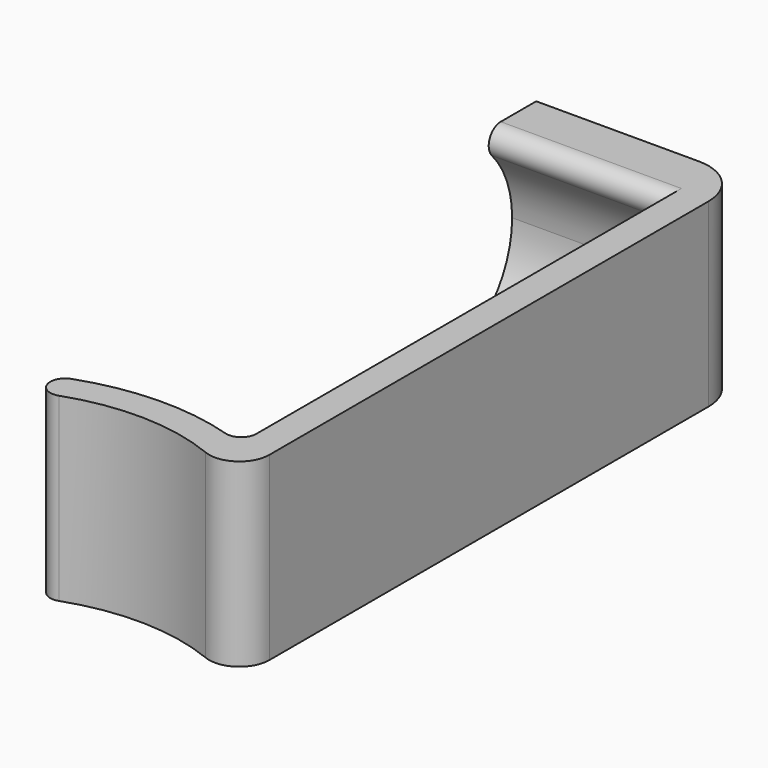
from build123d import *

# Parameters (mm, degrees)
F2_DEPTH    = 9.525
F3_DEPTH    = 19.05
F4_T1_DEPTH = 31.861787518
F5_R        = 5.08


# Not quite as in the source:
# - a fillet or chamfer that OpenCascade refuses, or shapes differently, is made with other operations: its cross-section is extruded or revolved along the edge and cut away or added


with BuildPart() as f2:
    # F0 (on Top) → F2 (new body, symmetric)
    with BuildSketch(Plane.XY):
        with BuildLine():
            Line((0, 3.175), (0, 0))
            Line((0, 0), (19.05, 0))
            Line((19.05, 0), (19.05, -57.5181780653))
            ThreePointArc((19.05, -57.5181780653), (18.4056155347, -58.7951625359), (16.9955882353, -59.0354617085))
            ThreePointArc((16.9955882353, -59.0354617085), (9.0004674941, -57.9174166081), (1.0583333333, -59.3646503438))
            ThreePointArc((1.0583333333, -59.3646503438), (0.2913116778, -59.944816145), (0, -60.8613596973))
            ThreePointArc((0, -60.8613596973), (0.6709564477, -62.1575480195), (2.1166666667, -62.3580690508))
            ThreePointArc((2.1166666667, -62.3580690508), (10.0201305345, -61.0925159656), (17.859375, -62.708873578))
            ThreePointArc((17.859375, -62.708873578), (20.8248789571, -62.3981407308), (22.225, -59.7655698035))
            Line((22.225, -59.7655698035), (22.225, 3.175))
            Line((22.225, 3.175), (0, 3.175))
        make_face()
    extrude(amount=F2_DEPTH, both=True)

    # F1 (on Right) → F3 (join, through all)
    with BuildSketch(Plane.YZ):
        with BuildLine():
            Line((-6.6244696296, -9.525), (0, -9.525))
            Line((0, -9.525), (0, 0))
            ThreePointArc((0, 0), (-1.8189392592, -5.8010607408), (-6.6244696296, -9.525))
        make_face()
        with BuildLine():
            ThreePointArc((-6.6244696296, 9.525), (-1.8189392592, 5.8010607408), (0, 0))
            Line((0, 0), (0, 9.525))
            Line((0, 9.525), (-6.6244696296, 9.525))
        make_face()
    extrude(amount=F3_DEPTH)

    # F4: fillet of radius 1.5875 on 2 edges, made by hand

    # F4_s2 → F4_t1 (cut)
    with BuildSketch(Plane.YZ.offset(-12.811787518)):
        with BuildLine():
            ThreePointArc((-1.4997546224, 9.525), (-2.9528486536, 8.5767761426), (-2.6700580518, 6.8648648649))
            ThreePointArc((-2.6700580518, 6.8648648649), (-4.4890794666, 8.4300806819), (-6.6244696296, 9.525))
            Line((-6.6244696296, 9.525), (-1.4997546224, 9.525))
        make_face()
        with BuildLine():
            ThreePointArc((-1.4997546224, -9.525), (-2.9528486536, -8.5767761426), (-2.6700580518, -6.8648648649))
            ThreePointArc((-2.6700580518, -6.8648648649), (-4.4890794666, -8.4300806819), (-6.6244696296, -9.525))
            Line((-6.6244696296, -9.525), (-1.4997546224, -9.525))
        make_face()
    extrude(amount=F4_T1_DEPTH, mode=Mode.SUBTRACT)

    # F5
    f5_edges = [f2.edges().sort_by_distance(p)[0] for p in [
        (22.225, 3.175, -4.7625),
        (22.225, 3.175, 4.7625),
    ]]
    fillet(f5_edges, radius=F5_R)


solid = f2.part
